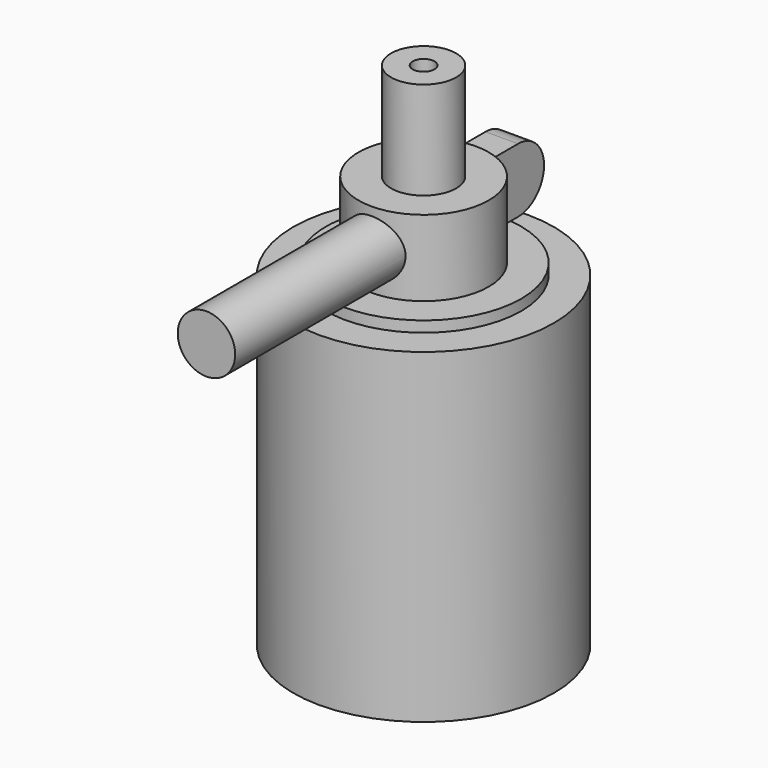
from build123d import *

# Parameters (mm, degrees)
F0_R         = 12
F1_DEPTH     = 30
F2_R         = 9
F3_DEPTH     = 1
F4_R         = 6
F5_DEPTH     = 7
F6_R         = 3
F7_DEPTH     = 9
F8_R         = 1
F9_DEPTH     = 25
F10_R        = 2.6468455099
F11_DEPTH    = 25
F12_W        = 3
F12_H        = 5.9210534014
F13_DEPTH    = 12
F14_T1_DEPTH = 18


# Not quite as in the source:
# - a fillet or chamfer that OpenCascade refuses, or shapes differently, is made with other operations: its cross-section is extruded or revolved along the edge and cut away or added


with BuildPart() as f1:
    # F0 (on Top) → F1 (new body)
    with BuildSketch(Plane.XY):
        Circle(F0_R)
    extrude(amount=F1_DEPTH)

    # F2 (on face) → F3 (join)
    with BuildSketch(Plane.XY.offset(30)):
        Circle(F2_R)
    extrude(amount=F3_DEPTH)

    # F4 (on face) → F5 (join)
    with BuildSketch(Plane.XY.offset(31)):
        Circle(F4_R)
    extrude(amount=F5_DEPTH)

    # F6 (on face) → F7 (join)
    with BuildSketch(Plane.XY.offset(38)):
        Circle(F6_R)
    extrude(amount=F7_DEPTH)

    # F8 (on face) → F9 (cut)
    with BuildSketch(Plane.XY.offset(47)):
        Circle(F8_R)
    extrude(amount=-F9_DEPTH, mode=Mode.SUBTRACT)

    # F10 (on Front) → F11 (join)
    with BuildSketch(Plane.XZ):
        with Locations((0, 34.5747359097)):
            Circle(F10_R)
    extrude(amount=F11_DEPTH)

    # F12 (on Front) → F13 (join)
    with BuildSketch(Plane.XZ):
        with Locations((0, 34.5066897571)):
            Rectangle(F12_W, F12_H)
    extrude(amount=-F13_DEPTH)

    # F14: fillet of radius 3 on 2 edges, made by hand

    # F14_s2 → F14_t1 (cut)
    with BuildSketch(Plane.YZ.offset(-9)):
        with BuildLine():
            ThreePointArc((9, 37.4672164578), (11.1213203436, 36.5885368014), (12, 34.4672164578))
            Line((12, 34.4672164578), (12, 37.4672164578))
            Line((12, 37.4672164578), (9, 37.4672164578))
        make_face()
        with BuildLine():
            ThreePointArc((9, 31.5461630564), (11.1213203436, 32.4248427128), (12, 34.5461630564))
            Line((12, 34.5461630564), (12, 31.5461630564))
            Line((12, 31.5461630564), (9, 31.5461630564))
        make_face()
    extrude(amount=F14_T1_DEPTH, mode=Mode.SUBTRACT)


solid = f1.part
